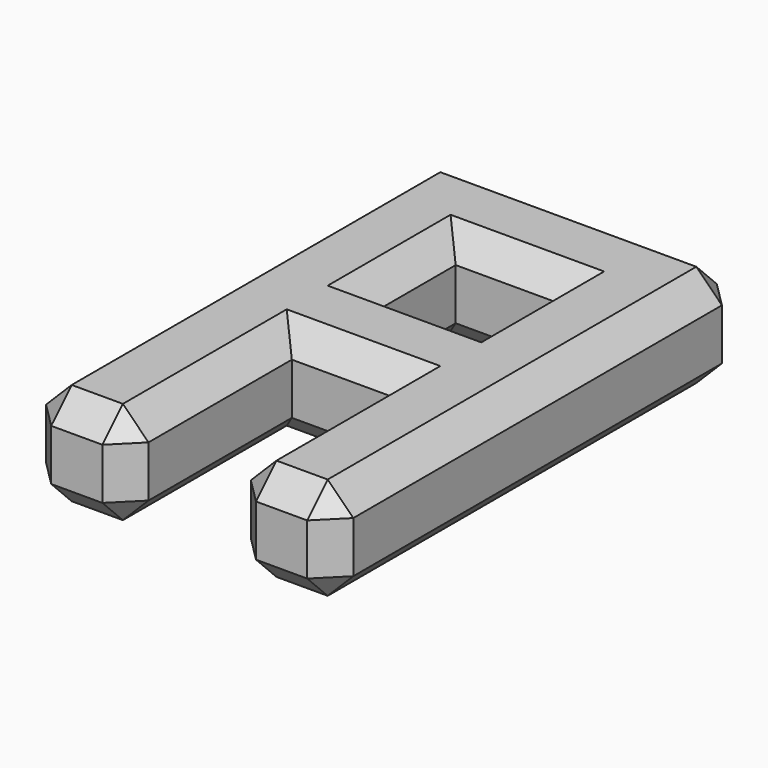
from build123d import *

# Parameters (mm, degrees)
F0_W     = 15.24
F0_H     = 25.4
F1_DEPTH = 5.08
F2_W     = 5.08
F2_H     = 5.08
F2_H_2   = 10.16
F3_DEPTH = 5.08
F4_SIZE  = 1.27


with BuildPart() as f1:
    # F0 (on Top) → F1 (new body)
    with BuildSketch(Plane.XY):
        Rectangle(F0_W, F0_H)
    extrude(amount=F1_DEPTH)

    # F2 (on face) → F3 (cut)
    with BuildSketch(Plane.XY.offset(5.08)):
        with Locations((0, 5.08)):
            Rectangle(F2_W, F2_H)
        with Locations((0, -7.62)):
            Rectangle(F2_W, F2_H_2)
    extrude(amount=-F3_DEPTH, mode=Mode.SUBTRACT)

    # F4
    f4_edges = [f1.edges().sort_by_distance(p)[0] for p in [
        (0, 7.62, 5.08),
        (0, 7.62, 0),
        (-2.54, 5.08, 5.08),
        (0, 2.54, 5.08),
        (2.54, 5.08, 5.08),
        (0, -2.54, 5.08),
        (-2.54, -7.62, 5.08),
        (2.54, -7.62, 5.08),
        (-7.62, 0, 5.08),
        (7.62, 0, 5.08),
        (0, 12.7, 5.08),
        (-5.08, -12.7, 5.08),
        (5.08, -12.7, 5.08),
        (-2.54, -12.7, 2.54),
        (2.54, -12.7, 2.54),
        (7.62, -12.7, 2.54),
        (-7.62, -12.7, 2.54),
        (-5.08, -12.7, 0),
        (5.08, -12.7, 0),
        (-7.62, 0, 0),
        (7.62, 0, 0),
        (-2.54, -7.62, 0),
        (2.54, -7.62, 0),
        (0, -2.54, 0),
        (0, 12.7, 0),
        (-2.54, 5.08, 0),
        (0, 2.54, 0),
        (2.54, 5.08, 0),
        (-7.62, 12.7, 2.54),
        (7.62, 12.7, 2.54),
    ]]
    chamfer(f4_edges, length=F4_SIZE)


solid = f1.part
